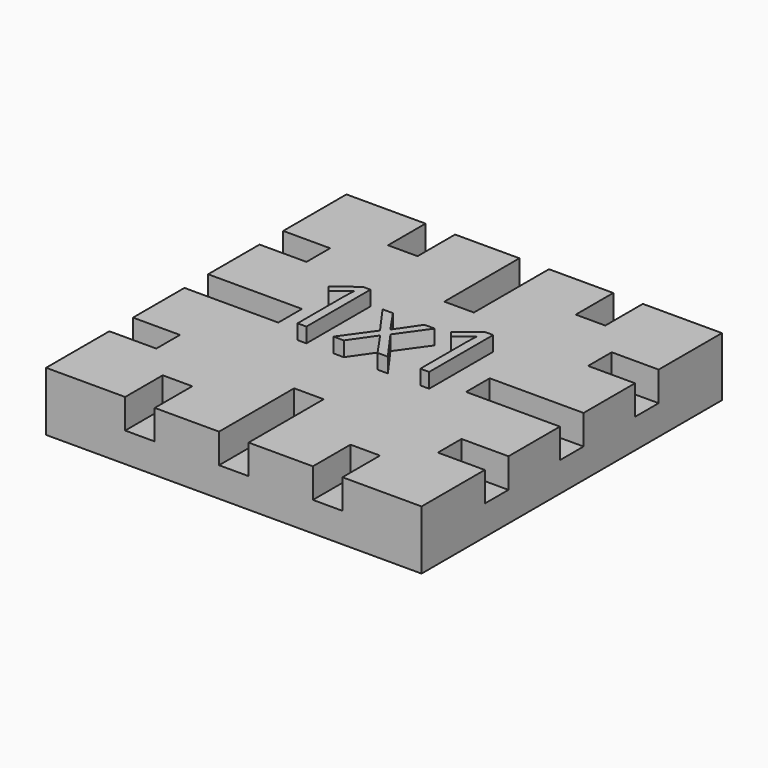
from build123d import *

# Parameters (mm, degrees)
F0_W         = 25.4
F0_H         = 25.4
F1_DEPTH     = 4
F2_W         = 2
F2_H         = 12.7
F2_H_2       = 6.35
F2_W_2       = 12.7
F2_H_3       = 2
F2_W_3       = 6.35
F3_DEPTH     = 2
F4_TEXT_SIZE = 7.5807313784
F5_DEPTH     = 1


# Not quite as in the source:
# - Text() gives the source's letters only with a copy of the font that has no kerning and outlines rounded to 1/6400 em; it was checked with that copy


with BuildPart() as f1:
    # F0 (on Top) → F1 (new body)
    with BuildSketch(Plane.XY):
        Rectangle(F0_W, F0_H)
    extrude(amount=F1_DEPTH)

    # F2 (on face) → F3 (cut)
    with BuildSketch(Plane.XY.offset(4)):
        with Locations((0, -12.7)):
            Rectangle(F2_W, F2_H)
        with Locations((6.35, -12.7)):
            Rectangle(F2_W, F2_H_2)
        with Locations((-6.35, -12.7)):
            Rectangle(F2_W, F2_H_2)
        with Locations((-12.7, 0)):
            Rectangle(F2_W_2, F2_H_3)
        with Locations((-12.7, 6.35)):
            Rectangle(F2_W_3, F2_H_3)
        with Locations((-12.7, -6.35)):
            Rectangle(F2_W_3, F2_H_3)
        with Locations((0, 12.7)):
            Rectangle(F2_W, F2_H)
        with Locations((-6.35, 12.7)):
            Rectangle(F2_W, F2_H_2)
        with Locations((6.35, 12.7)):
            Rectangle(F2_W, F2_H_2)
        with Locations((12.7, 0)):
            Rectangle(F2_W_2, F2_H_3)
        with Locations((12.7, -6.35)):
            Rectangle(F2_W_3, F2_H_3)
        with Locations((12.7, 6.35)):
            Rectangle(F2_W_3, F2_H_3)
    extrude(amount=-F3_DEPTH, mode=Mode.SUBTRACT)

    # F4 (on face) → F5 (join)
    with BuildSketch(Plane.XY.offset(4)):
        with Locations((-6.35, -1.9321369316)):
            Text('1x1', F4_TEXT_SIZE, font='Open Sans', text_align=(TextAlign.LEFT, TextAlign.BOTTOM))
    extrude(amount=F5_DEPTH)


solid = f1.part
